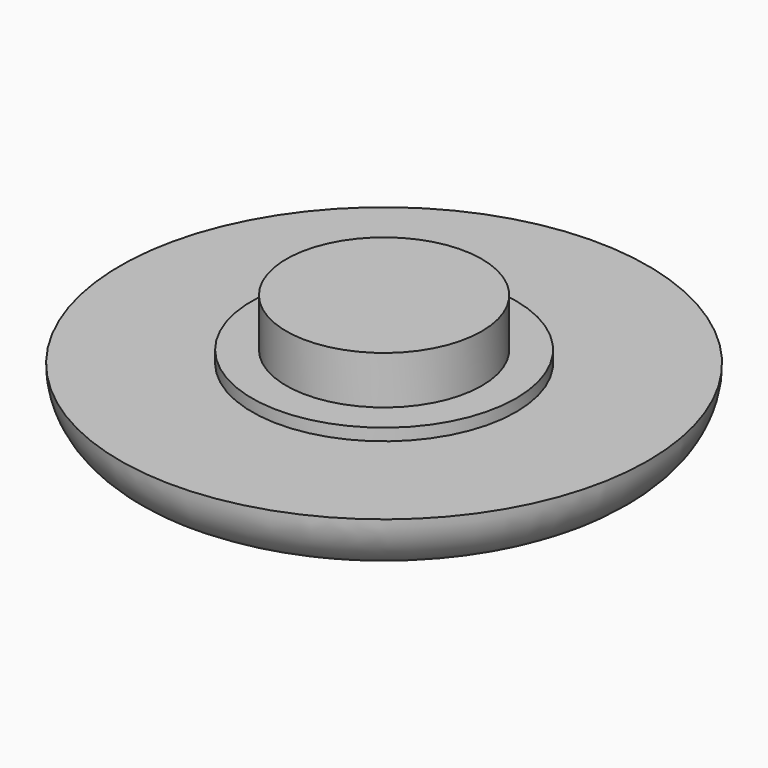
from build123d import *

# Parameters (mm, degrees)
F0_R     = 11
F0_R_2   = 5.5
F1_DEPTH = 2.5
F0_R_3   = 4.075
F2_DEPTH = 3
F3_DEPTH = 5
F4_R     = 2.49999


# Not quite as in the source:
# - a fillet or chamfer is up to 0.001 mm smaller than in the source, because OpenCascade refuses the exact size


with BuildPart() as f1:
    # F0 (on Top) → F1 (new body)
    with BuildSketch(Plane.XY):
        with Locations((-41.2729866803, 41.5038391948)):
            Circle(F0_R)
        with Locations((-41.2729866803, 41.5038391948)):
            Circle(F0_R_2, mode=Mode.SUBTRACT)
    extrude(amount=F1_DEPTH)

    # F0 (on Top) → F2 (join)
    with BuildSketch(Plane.XY):
        with Locations((-41.2729866803, 41.5038391948)):
            Circle(F0_R_2)
        with Locations((-41.2729866803, 41.5038391948)):
            Circle(F0_R_3, mode=Mode.SUBTRACT)
    extrude(amount=F2_DEPTH)

    # F0 (on Top) → F3 (join)
    with BuildSketch(Plane.XY):
        with Locations((-41.2729866803, 41.5038391948)):
            Circle(F0_R_3)
    extrude(amount=F3_DEPTH)

    # F4 (radius 2.5 in the source; OpenCascade refuses exactly that, so slightly less here)
    f4_edges = [f1.edges().sort_by_distance(p)[0] for p in [
        (-52.272987, 41.503839, 0),
    ]]
    fillet(f4_edges, radius=F4_R)


solid = f1.part
